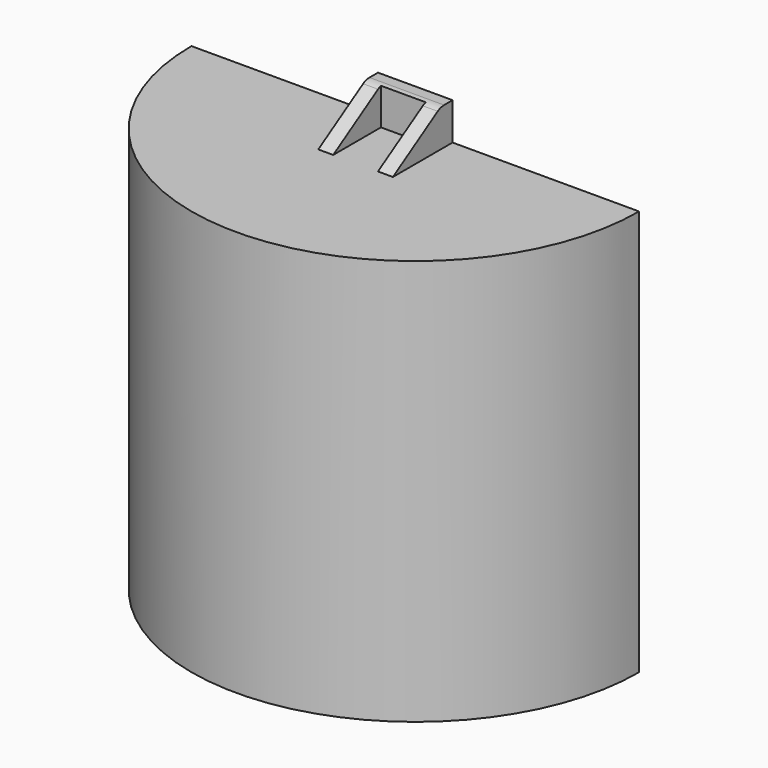
from build123d import *

# Parameters (mm, degrees)
F1_DEPTH     = 4.7625
F3_DEPTH     = 127
F5_DEPTH     = 6.35
F7_DEPTH     = 12.7
F9_DEPTH     = 5.08
F10_T1_DEPTH = 22.563097962
F10_T3_DEPTH = 22.563097962


# Not quite as in the source:
# - a fillet or chamfer that OpenCascade refuses, or shapes differently, is made with other operations: its cross-section is extruded or revolved along the edge and cut away or added
# - a length typed as a fraction of an inch, garbled in the dataset ("3 / 203.2 mm" for 3/8 in), is restored
# - a pattern or mirror of a feature is missing from the dataset's text; its kind, count and spacing are read off the source's solid


with BuildPart() as f1:
    # F0 (on Top) → F1 (new body)
    with BuildSketch(Plane.XY):
        with BuildLine():
            ThreePointArc((-76.2, 0), (0, -76.2), (76.2, 0))
            Line((76.2, 0), (67.31, 0))
            Line((67.31, 0), (67.31, -12.7))
            Line((67.31, -12.7), (-67.31, -12.7))
            Line((-67.31, -12.7), (-67.31, 0))
            Line((-67.31, 0), (-76.2, 0))
        make_face()
    extrude(amount=F1_DEPTH)

    # F2 (on face) → F3 (join)
    with BuildSketch(Plane.XY.offset(4.7625)):
        with BuildLine():
            Line((-67.31, 0), (-76.2, 0))
            ThreePointArc((-76.2, 0), (0, -76.2), (76.2, 0))
            Line((76.2, 0), (67.31, 0))
            ThreePointArc((67.31, 0), (0, -67.31), (-67.31, 0))
        make_face()
    extrude(amount=F3_DEPTH)

    # F4 (on face) → F5 (join)
    with BuildSketch(Plane.XY.offset(131.7625)):
        with BuildLine():
            Line((76.2, 0), (-76.2, 0))
            ThreePointArc((-76.2, 0), (0, -76.2), (76.2, 0))
        make_face()
    extrude(amount=F5_DEPTH)

    # F6 (on face) → F7 (join)
    with BuildSketch(Plane.XY.offset(138.1125)):
        Polygon((12.7, 0), (0, 0), (-12.7, 0), (-12.7, -5.08), (0, -5.08), (12.7, -5.08), align=None)
    extrude(amount=F7_DEPTH)

    # F8 (on face) → F9 (join)
    with BuildSketch(Plane.YZ.offset(12.7)):
        Polygon((-5.08, 150.8125), (-25.4, 138.1125), (-5.08, 138.1125), align=None)
    f9 = extrude(amount=-F9_DEPTH)

    # F9_copies: F9 across plane
    add(f9.mirror(Plane(origin=(0, 0, 0), x_dir=(0, 0, -1), z_dir=(-1, 0, 0))))

    # F10: fillet of radius 5.08 on 2 edges, made by hand

    # F10_s2 → F10_t1 (cut)
    with BuildSketch(Plane.YZ.offset(-21.441548981)):
        with BuildLine():
            ThreePointArc((-6.315469785, 150.0403313843), (-5.0235423361, 150.6156436305), (-3.6230751698, 150.8125))
            Line((-3.6230751698, 150.8125), (-3.6230751698, 150.9141))
            Line((-3.6230751698, 150.9141), (-5.1091384966, 150.9141))
            Line((-5.1091384966, 150.9141), (-6.3693176774, 150.126488012))
            Line((-6.3693176774, 150.126488012), (-6.315469785, 150.0403313843))
        make_face()
    extrude(amount=F10_T1_DEPTH, mode=Mode.SUBTRACT)

    # F10_s4 → F10_t3 (cut)
    with BuildSketch(Plane.YZ.offset(-1.121548981)):
        with BuildLine():
            ThreePointArc((-3.6230751698, 150.8125), (-5.0235423361, 150.6156436305), (-6.315469785, 150.0403313843))
            Line((-6.315469785, 150.0403313843), (-6.3693176774, 150.126488012))
            Line((-6.3693176774, 150.126488012), (-5.1091384966, 150.9141))
            Line((-5.1091384966, 150.9141), (-3.6230751698, 150.9141))
            Line((-3.6230751698, 150.9141), (-3.6230751698, 150.8125))
        make_face()
    extrude(amount=F10_T3_DEPTH, mode=Mode.SUBTRACT)


solid = f1.part
